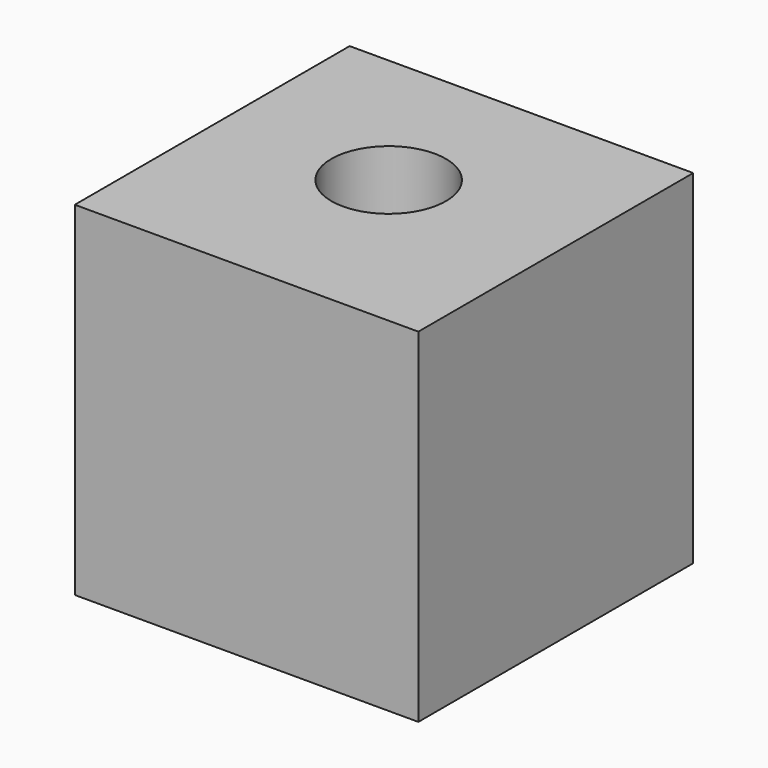
from build123d import *

# Parameters (mm, degrees)
F0_W     = 76.2
F0_H     = 76.2
F1_DEPTH = 76.2
F7_D     = 25.4


# Not quite as in the source:
# - the program builds the solid bodies; features that only make, move or delete a surface that nothing else refers to are left out


with BuildPart() as f1:
    # F0 (on Front) → F1 (new body)
    with BuildSketch(Plane.XZ):
        with Locations((-1.327181235, 7.6158734726)):
            Rectangle(F0_W, F0_H)
    extrude(amount=F1_DEPTH)

    # F7 (through all)
    with Locations(Plane.XY.offset(45.7158734726)):
        with Locations((-2.7743626852, -34.9938422441)):
            Hole(F7_D / 2)


solid = f1.part
